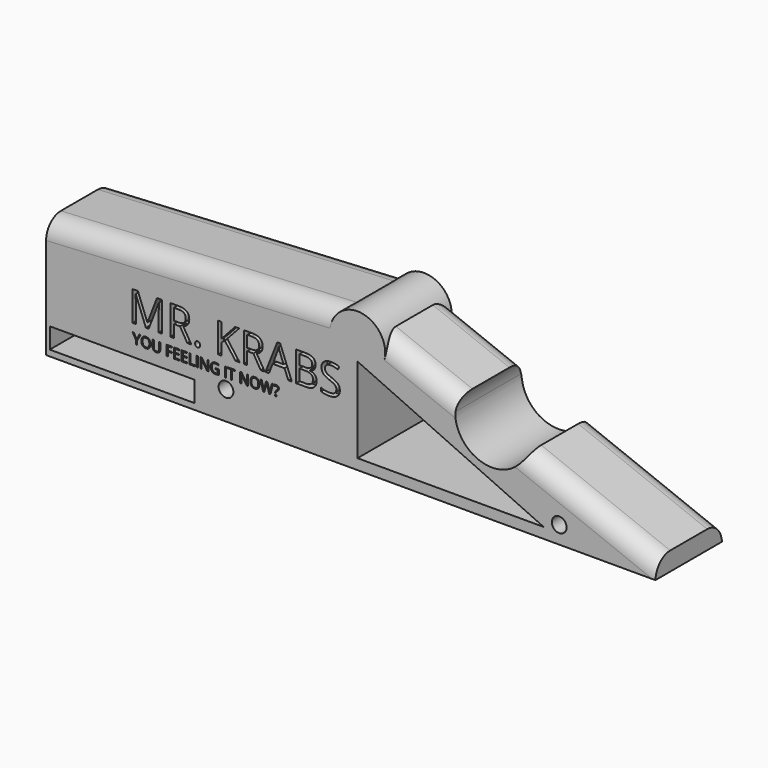
from build123d import *

# Parameters (mm, degrees)
F1_DEPTH      = 40
F2_R          = 2
F3_DEPTH      = 40.001
F4_DEPTH      = 17.5
F5_R          = 5
F6_DEPTH      = 60
F8_DEPTH      = 22.501
F10_DEPTH     = 22.5
F11_R         = 5
F12_R         = 5
F13_TEXT_SIZE = 11.2890356427
F14_DEPTH     = 2
F16_R         = 2
F17_DEPTH     = 22.5010001
F19_DEPTH     = 22.5010001
F20_TEXT_SIZE = 3.7843646068
F21_DEPTH     = 2.5
F22_W         = 39.1012355685
F22_H         = 5.5582467467
F23_DEPTH     = 22.5010001


# Not quite as in the source:
# - Text() gives the source's letters only with a copy of the font that has no kerning and outlines rounded to 1/6400 em; it was checked with that copy


with BuildPart() as f1:
    # F0 (on Front) → F1 (new body)
    with BuildSketch(Plane.XZ):
        Polygon((-84.199729269, 0), (-84.199729269, -32.2991868854), (80.534145236, -32.2991868854), (80.534145236, -27.2749941796), (0, 4.4790389948), align=None)
    extrude(amount=F1_DEPTH)

    # F2 (on face) → F3 (cut, through all)
    with BuildSketch(Plane.XZ.offset(40)):
        with Locations((-35.5611145496, -24.6386155486)):
            Circle(F2_R)
        with Locations((174.3349283934, -24.6386155486)):
            Circle(F2_R)
    extrude(amount=-F3_DEPTH, mode=Mode.SUBTRACT)

    # F2 (on face) → F4 (cut)
    with BuildSketch(Plane.XZ.offset(40)):
        Polygon((80.534145236, -32.2991868854), (80.534145236, -27.2749941796), (0, 4.4790389948), (-84.199729269, 0), (-84.199729269, -32.2991868854), align=None)
        with Locations((-35.5611145496, -24.6386155486)):
            Circle(F2_R, mode=Mode.SUBTRACT)
    extrude(amount=-F4_DEPTH, mode=Mode.SUBTRACT)

    # F5 (on face) → F6 (cut)
    with BuildSketch(Plane(origin=(-84.199729269, 0, 0), x_dir=(0, -1, 0), z_dir=(-1, 0, 0))):
        with Locations((11.25, -16.1495934427)):
            Circle(F5_R)
    extrude(amount=-F6_DEPTH, mode=Mode.SUBTRACT)

    # F7 (on face) → F8 (cut, through all)
    with BuildSketch(Plane(origin=(0, 0, 0), x_dir=(-1, 0, 0), z_dir=(0, 1, 0))):
        with BuildLine():
            ThreePointArc((-45.6708906422, -13.5286641019), (-34.5010623989, -19.6847683032), (-26.3679283029, -9.8605730844))
            ThreePointArc((-26.3679283029, -9.8605730844), (-26.5437330841, -7.9937071805), (-27.0649659635, -6.1924820669))
            Line((-27.0649659635, -6.1924820669), (-45.6708906422, -13.5286641019))
        make_face()
    extrude(amount=-F8_DEPTH, mode=Mode.SUBTRACT)

    # F9 (on face) → F10 (join)
    with BuildSketch(Plane(origin=(0, 0, 0), x_dir=(-1, 0, 0), z_dir=(0, 1, 0))):
        with BuildLine():
            Line((0, 4.4790389948), (4.151824079, 4.2581810168))
            ThreePointArc((4.151824079, 4.2581810168), (-1.5958657894, 5.3404413252), (-6.3730642438, 1.9661856848))
            Line((-6.3730642438, 1.9661856848), (0, 4.4790389948))
        make_face()
    extrude(amount=-F10_DEPTH)

    # F11
    f11_edges = [f1.edges().sort_by_distance(p)[0] for p in [
        (-44.175777, -22.5, 2.129091),
        (-44.175777, 0, 2.129091),
    ]]
    fillet(f11_edges, radius=F11_R)

    # F12
    f12_edges = [f1.edges().sort_by_distance(p)[0] for p in [
        (63.102518, -22.5, -20.401829),
        (63.102518, 0, -20.401829),
        (16.719015, 0, -2.113148),
        (16.719015, -22.5, -2.113148),
    ]]
    fillet(f12_edges, radius=F12_R)

    # F13 (on face) → F14 (cut)
    with BuildSketch(Plane.XZ.offset(22.5)):
        with Locations((-61.8980489671, -17.0245580375)):
            Text('MR. KRABS', F13_TEXT_SIZE, font='Open Sans', text_align=(TextAlign.LEFT, TextAlign.BOTTOM))
    extrude(amount=-F14_DEPTH, mode=Mode.SUBTRACT)

    # F16 (on face) → F17 (cut, through all)
    with BuildSketch(Plane(origin=(0, 0, 0), x_dir=(-1, 0, 0), z_dir=(0, 1, 0))):
        with Locations((-54.531738162, -27.5621432811)):
            Circle(F16_R)
    extrude(amount=-F17_DEPTH, mode=Mode.SUBTRACT)

    # F18 (on face) → F19 (cut, through all)
    with BuildSketch(Plane.XZ.offset(22.5)):
        Polygon((50.3553450108, -29.4556692243), (0, -6.4328624867), (0, -29.4556692243), align=None)
    extrude(amount=-F19_DEPTH, mode=Mode.SUBTRACT)

    # F20 (on face) → F21 (cut)
    with BuildSketch(Plane.XZ.offset(22.5)):
        with Locations((-60.7903123447, -21.9100322574)):
            Text('YOU FEELING IT NOW?', F20_TEXT_SIZE, font='Open Sans', text_align=(TextAlign.LEFT, TextAlign.BOTTOM))
    extrude(amount=-F21_DEPTH, mode=Mode.SUBTRACT)

    # F22 (on face) → F23 (cut, through all)
    with BuildSketch(Plane.XZ.offset(22.5)):
        with Locations((-63.6528320611, -27.8913630173)):
            Rectangle(F22_W, F22_H)
    extrude(amount=-F23_DEPTH, mode=Mode.SUBTRACT)


solid = f1.part
